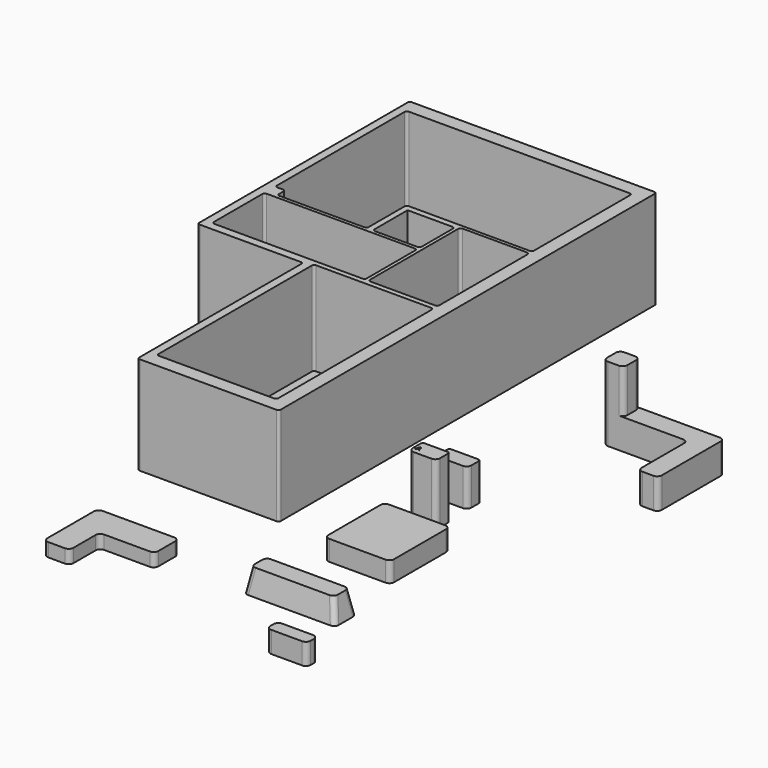
from build123d import *

# Parameters (mm, degrees)
F1_W          = 5.7142857143
F1_H          = 5.8571428571
F1_W_2        = 50.5714285714
F1_W_3        = 3.4285714286
F1_W_4        = 95.2142857143
F1_H_2        = 3.4285714286
F1_W_5        = 4.2857142857
F1_H_3        = 4.2857142857
F2_DEPTH      = 41.4285714286
F1_W_6        = 29.2571428571
F1_H_4        = 48.5
F1_W_7        = 19.9
F1_H_5        = 18.4142857143
F1_H_6        = 82.8571428571
F3_DEPTH      = 2
F4_R          = 1
F5_R          = 1
F6_W          = 13.2857142857
F6_H          = 6.8571428571
F7_DEPTH      = 15.7142857143
F8_R          = 2
F9_R          = 1
F10_TEXT_SIZE = 2.7525218116
F11_DEPTH     = 0.4
F12_W         = 11.5714285714
F12_H         = 7.1428571429
F13_DEPTH     = 25.7142857143
F14_R         = 2
F15_R         = 1
F16_TEXT_SIZE = 2.7248175908
F17_DEPTH     = 0.4
F18_W         = 27.7142857143
F18_H         = 31.4285714286
F19_DEPTH     = 8.5714285714
F20_R         = 2
F21_W         = 38.5714285714
F21_H         = 11.4285714286
F22_DEPTH     = 10
F22_TAPER     = 10
F23_R         = 2
F25_DEPTH     = 5.7142857143
F26_R         = 2
F28_DEPTH     = 12.8571428571
F27_W         = 8.5714285714
F27_H         = 8.5714285714
F29_DEPTH     = 31.4285714286
F30_R         = 2
F31_W         = 17
F31_H         = 5.7142857143
F32_DEPTH     = 9
F33_R         = 2


# Not quite as in the source:
# - Text() gives the source's letters only with a copy of the font that has no kerning and outlines rounded to 1/6400 em; it was checked with that copy


with BuildPart() as f2:
    # F1 (on Top) → F2 (new body)
    with BuildSketch(Plane.XY):
        with Locations((-2.8571428571, 2.9285714286)):
            Rectangle(F1_W, F1_H)
        with Locations((-31, 2.9285714286)):
            Rectangle(F1_W_2, F1_H)
        Polygon((-5.7142857143, 5.8571428571), (0, 5.8571428571), (0, 193.5), (-5.7142857143, 193.5), (-5.7142857143, 140.7857142857), (-5.7142857143, 139.3571428571), (-5.7142857143, 90.8571428571), (-5.7142857143, 88.7142857143), align=None)
        with Locations((-58, 2.9285714286)):
            Rectangle(F1_W_3, F1_H)
        with Locations((-2.8571428571, 196.4285714286)):
            Rectangle(F1_W, F1_H)
        Polygon((-59.7142857143, 5.8571428571), (-56.2857142857, 5.8571428571), (-56.2857142857, 88.7142857143), (-56.2857142857, 90.8571428571), (-100.9285714286, 90.8571428571), (-100.9285714286, 87.4285714286), (-59.7142857143, 87.4285714286), align=None)
        with Locations((-53.3214285714, 196.4285714286)):
            Rectangle(F1_W_4, F1_H)
        Polygon((-100.9285714286, 124.1571428571), (-100.9285714286, 193.5), (-104.3571428571, 193.5), (-104.3571428571, 90.8571428571), (-100.9285714286, 90.8571428571), (-100.9285714286, 118.4428571429), (-100.9285714286, 119.8714285714), align=None)
        with Locations((-102.6428571429, 196.4285714286)):
            Rectangle(F1_W_3, F1_H)
        with Locations((-102.6428571429, 89.1428571429)):
            Rectangle(F1_W_3, F1_H_2)
        Polygon((-36.4, 138.2857142857), (-36.4, 140.7857142857), (-58.8, 140.7857142857), (-58.8, 119.8714285714), (-56.3, 119.8714285714), (-56.3, 138.2857142857), align=None)
        Polygon((-5.7142857143, 139.3571428571), (-5.7142857143, 140.7857142857), (-36.4, 140.7857142857), (-36.4, 138.2857142857), (-36.4, 119.8714285714), (-36.4, 118.4428571429), (-36.4, 90.8571428571), (-34.9714285714, 90.8571428571), (-34.9714285714, 139.3571428571), align=None)
        Polygon((-56.2857142857, 88.7142857143), (-5.7142857143, 88.7142857143), (-5.7142857143, 90.8571428571), (-34.9714285714, 90.8571428571), (-36.4, 90.8571428571), (-56.2857142857, 90.8571428571), align=None)
        Polygon((-58.8, 118.4428571429), (-36.4, 118.4428571429), (-36.4, 119.8714285714), (-56.3, 119.8714285714), (-58.8, 119.8714285714), align=None)
        with Locations((-98.7857142857, 122.0142857143)):
            Rectangle(F1_W_5, F1_H_3)
        Polygon((-96.6428571429, 119.8714285714), (-100.9285714286, 119.8714285714), (-100.9285714286, 118.4428571429), (-58.8, 118.4428571429), (-58.8, 119.8714285714), align=None)
    extrude(amount=F2_DEPTH)

    # F1 (on Top) → F3 (join)
    with BuildSketch(Plane.XY):
        with Locations((-2.8571428571, 2.9285714286)):
            Rectangle(F1_W, F1_H)
        with Locations((-31, 2.9285714286)):
            Rectangle(F1_W_2, F1_H)
        Polygon((-5.7142857143, 5.8571428571), (0, 5.8571428571), (0, 193.5), (-5.7142857143, 193.5), (-5.7142857143, 140.7857142857), (-5.7142857143, 139.3571428571), (-5.7142857143, 90.8571428571), (-5.7142857143, 88.7142857143), align=None)
        with Locations((-58, 2.9285714286)):
            Rectangle(F1_W_3, F1_H)
        with Locations((-2.8571428571, 196.4285714286)):
            Rectangle(F1_W, F1_H)
        Polygon((-59.7142857143, 5.8571428571), (-56.2857142857, 5.8571428571), (-56.2857142857, 88.7142857143), (-56.2857142857, 90.8571428571), (-100.9285714286, 90.8571428571), (-100.9285714286, 87.4285714286), (-59.7142857143, 87.4285714286), align=None)
        with Locations((-53.3214285714, 196.4285714286)):
            Rectangle(F1_W_4, F1_H)
        Polygon((-100.9285714286, 124.1571428571), (-100.9285714286, 193.5), (-104.3571428571, 193.5), (-104.3571428571, 90.8571428571), (-100.9285714286, 90.8571428571), (-100.9285714286, 118.4428571429), (-100.9285714286, 119.8714285714), align=None)
        with Locations((-102.6428571429, 196.4285714286)):
            Rectangle(F1_W_3, F1_H)
        with Locations((-102.6428571429, 89.1428571429)):
            Rectangle(F1_W_3, F1_H_2)
        Polygon((-5.7142857143, 140.7857142857), (-5.7142857143, 193.5), (-100.9285714286, 193.5), (-100.9285714286, 124.1571428571), (-96.6428571429, 124.1571428571), (-96.6428571429, 119.8714285714), (-58.8, 119.8714285714), (-58.8, 140.7857142857), (-36.4, 140.7857142857), align=None)
        Polygon((-36.4, 138.2857142857), (-36.4, 140.7857142857), (-58.8, 140.7857142857), (-58.8, 119.8714285714), (-56.3, 119.8714285714), (-56.3, 138.2857142857), align=None)
        with Locations((-20.3428571429, 115.1071428571)):
            Rectangle(F1_W_6, F1_H_4)
        Polygon((-100.9285714286, 90.8571428571), (-56.2857142857, 90.8571428571), (-36.4, 90.8571428571), (-36.4, 118.4428571429), (-58.8, 118.4428571429), (-100.9285714286, 118.4428571429), align=None)
        with Locations((-46.35, 129.0785714286)):
            Rectangle(F1_W_7, F1_H_5)
        with Locations((-31, 47.2857142857)):
            Rectangle(F1_W_2, F1_H_6)
        Polygon((-56.2857142857, 88.7142857143), (-5.7142857143, 88.7142857143), (-5.7142857143, 90.8571428571), (-34.9714285714, 90.8571428571), (-36.4, 90.8571428571), (-56.2857142857, 90.8571428571), align=None)
        Polygon((-5.7142857143, 139.3571428571), (-5.7142857143, 140.7857142857), (-36.4, 140.7857142857), (-36.4, 138.2857142857), (-36.4, 119.8714285714), (-36.4, 118.4428571429), (-36.4, 90.8571428571), (-34.9714285714, 90.8571428571), (-34.9714285714, 139.3571428571), align=None)
        Polygon((-58.8, 118.4428571429), (-36.4, 118.4428571429), (-36.4, 119.8714285714), (-56.3, 119.8714285714), (-58.8, 119.8714285714), align=None)
        Polygon((-96.6428571429, 119.8714285714), (-100.9285714286, 119.8714285714), (-100.9285714286, 118.4428571429), (-58.8, 118.4428571429), (-58.8, 119.8714285714), align=None)
        with Locations((-98.7857142857, 122.0142857143)):
            Rectangle(F1_W_5, F1_H_3)
    extrude(amount=F3_DEPTH)

    # F4
    f4_edges = [f2.edges().sort_by_distance(p)[0] for p in [
        (-100.928571, 193.5, 21.714286),
        (-100.928571, 124.157143, 21.714286),
        (-96.642857, 124.157143, 21.714286),
        (-96.642857, 119.871429, 21.714286),
        (-58.8, 119.871429, 21.714286),
        (-58.8, 140.785714, 21.714286),
        (-5.714286, 140.785714, 21.714286),
        (-5.714286, 193.5, 21.714286),
        (-36.4, 138.285714, 21.714286),
        (-56.3, 119.871429, 21.714286),
        (-36.4, 119.871429, 21.714286),
        (-34.971429, 139.357143, 21.714286),
        (-5.714286, 90.857143, 21.714286),
        (-34.971429, 90.857143, 21.714286),
        (-36.4, 118.442857, 21.714286),
        (-100.928571, 90.857143, 21.714286),
        (-36.4, 90.857143, 21.714286),
        (-5.714286, 88.714286, 21.714286),
        (-56.285714, 88.714286, 21.714286),
        (-56.285714, 5.857143, 21.714286),
        (-5.714286, 5.857143, 21.714286),
        (-5.714286, 139.357143, 21.714286),
        (-100.928571, 118.442857, 21.714286),
    ]]
    fillet(f4_edges, radius=F4_R)

    # F5
    f5_edges = [f2.edges().sort_by_distance(p)[0] for p in [
        (0, 0, 20.714286),
        (-59.714286, 0, 20.714286),
        (-59.714286, 87.428571, 20.714286),
        (-104.357143, 87.428571, 20.714286),
        (-104.357143, 199.357143, 20.714286),
        (0, 199.357143, 20.714286),
    ]]
    fillet(f5_edges, radius=F5_R)


with BuildPart() as f7:
    # F6 (on Top) → F7 (new body)
    with BuildSketch(Plane.XY):
        with Locations((36.4548806101, 49.1182368736)):
            Rectangle(F6_W, F6_H)
    extrude(amount=F7_DEPTH)

    # F8
    f8_edges = [f7.edges().sort_by_distance(p)[0] for p in [
        (29.812023, 45.689665, 7.857143),
        (43.097738, 45.689665, 7.857143),
    ]]
    fillet(f8_edges, radius=F8_R)

    # F9
    f9_edges = [f7.edges().sort_by_distance(p)[0] for p in [
        (43.097738, 52.546808, 7.857143),
        (29.812023, 52.546808, 7.857143),
    ]]
    fillet(f9_edges, radius=F9_R)

    # F10 (on face) → F11 (cut)
    with BuildSketch(Plane.XY.offset(15.7142857143)):
        with Locations((30.4349511862, 47.6364211693)):
            Text('K', F10_TEXT_SIZE, font='Open Sans', font_style=FontStyle.BOLD, text_align=(TextAlign.LEFT, TextAlign.BOTTOM))
    extrude(amount=-F11_DEPTH, mode=Mode.SUBTRACT)


with BuildPart() as f13:
    # F12 (on Top) → F13 (new body)
    with BuildSketch(Plane.XY):
        with Locations((38.0404666066, 31.8159611196)):
            Rectangle(F12_W, F12_H)
    extrude(amount=F13_DEPTH)

    # F14
    f14_edges = [f13.edges().sort_by_distance(p)[0] for p in [
        (32.254752, 28.244533, 12.857143),
        (43.826181, 28.244533, 12.857143),
    ]]
    fillet(f14_edges, radius=F14_R)

    # F15
    f15_edges = [f13.edges().sort_by_distance(p)[0] for p in [
        (43.826181, 35.38739, 12.857143),
        (32.254752, 35.38739, 12.857143),
    ]]
    fillet(f15_edges, radius=F15_R)

    # F16 (on face) → F17 (cut)
    with BuildSketch(Plane.XY.offset(25.7142857143)):
        with Locations((33.0834686756, 30.3540924542)):
            Text('A', F16_TEXT_SIZE, font='Open Sans', font_style=FontStyle.BOLD, text_align=(TextAlign.LEFT, TextAlign.BOTTOM))
    extrude(amount=-F17_DEPTH, mode=Mode.SUBTRACT)


with BuildPart() as f19:
    # F18 (on Top) → F19 (new body)
    with BuildSketch(Plane.XY):
        with Locations((42.609273456, 3.9195903868)):
            Rectangle(F18_W, F18_H)
    extrude(amount=F19_DEPTH)

    # F20
    f20_edges = [f19.edges().sort_by_distance(p)[0] for p in [
        (28.752131, -11.794695, 4.285714),
        (56.466416, -11.794695, 4.285714),
        (56.466416, 19.633876, 4.285714),
        (28.752131, 19.633876, 4.285714),
    ]]
    fillet(f20_edges, radius=F20_R)


with BuildPart() as f22:
    # F21 (on Top) → F22 (new body)
    with BuildSketch(Plane.XY):
        with Locations((42.0146109536, -41.3059583297)):
            Rectangle(F21_W, F21_H)
    extrude(amount=F22_DEPTH, taper=F22_TAPER)

    # F23
    f23_edges = [f22.edges().sort_by_distance(p)[0] for p in [
        (60.41869, -46.138609, 5),
        (23.610532, -46.138609, 5),
        (60.41869, -36.473308, 5.000003),
        (23.610532, -36.473308, 5),
    ]]
    fillet(f23_edges, radius=F23_R)


with BuildPart() as f25:
    # F24 (on Top) → F25 (new body)
    with BuildSketch(Plane.XY):
        Polygon((-11.3080516549, -38.6351870822), (-45.5937659406, -38.6351870822), (-45.5937659406, -67.2066156536), (-34.5937659406, -67.2066156536), (-34.5937659406, -51.4923299393), (-11.3080516549, -51.4923299393), align=None)
    extrude(amount=F25_DEPTH)

    # F26
    f26_edges = [f25.edges().sort_by_distance(p)[0] for p in [
        (-34.593766, -67.206616, 2.857143),
        (-45.593766, -67.206616, 2.857143),
        (-11.308052, -51.49233, 2.857143),
        (-11.308052, -38.635187, 2.857143),
        (-45.593766, -38.635187, 2.857143),
        (-34.593766, -51.49233, 2.857143),
    ]]
    fillet(f26_edges, radius=F26_R)


with BuildPart() as f28:
    # F27 (on Top) → F28 (new body)
    with BuildSketch(Plane.XY):
        Polygon((93.1343779128, 118.7056894728), (57.4200921985, 118.7056894728), (57.4200921985, 110.1342609013), (84.5629493413, 110.1342609013), (84.5629493413, 83.7056894728), (93.1343779128, 83.7056894728), align=None)
    extrude(amount=F28_DEPTH)

    # F27 (on Top) → F29 (join)
    with BuildSketch(Plane.XY):
        with Locations((53.1343779128, 114.4199751871)):
            Rectangle(F27_W, F27_H)
    extrude(amount=F29_DEPTH)

    # F30
    f30_edges = [f28.edges().sort_by_distance(p)[0] for p in [
        (48.848664, 110.134261, 15.714286),
        (84.562949, 110.134261, 6.428571),
        (84.562949, 83.705689, 6.428571),
        (93.134378, 83.705689, 6.428571),
        (93.134378, 118.705689, 6.428571),
        (48.848664, 118.705689, 15.714286),
        (57.420092, 110.134261, 22.142857),
        (57.420092, 118.705689, 22.142857),
    ]]
    fillet(f30_edges, radius=F30_R)


with BuildPart() as f32:
    # F31 (on Top) → F32 (new body)
    with BuildSketch(Plane.XY):
        with Locations((63.3983332664, -72.2702120298)):
            Rectangle(F31_W, F31_H)
    extrude(amount=F32_DEPTH)

    # F33
    f33_edges = [f32.edges().sort_by_distance(p)[0] for p in [
        (71.898333, -75.127355, 4.5),
        (54.898333, -75.127355, 4.5),
        (71.898333, -69.413069, 4.5),
        (54.898333, -69.413069, 4.5),
    ]]
    fillet(f33_edges, radius=F33_R)


solid = Compound([f2.part, f7.part, f13.part, f19.part, f22.part, f25.part, f28.part, f32.part])
